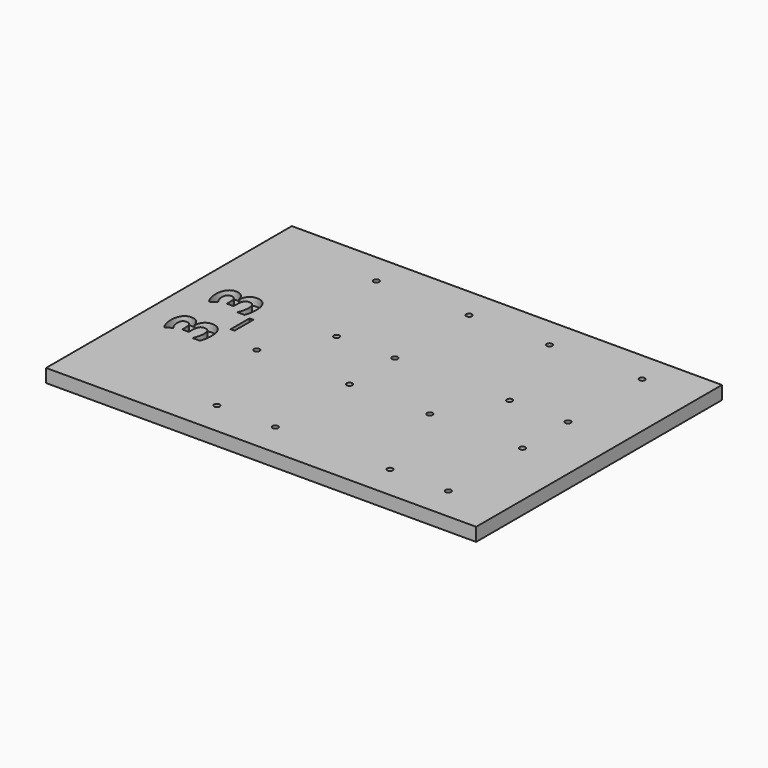
from build123d import *

# Parameters (mm, degrees)
F0_W         = 84
F0_H         = 60
F1_DEPTH     = 2.6
F2_TEXT_SIZE = 11.1111111111
F3_DEPTH     = 1.5
F4_R         = 0.55
F5_DEPTH     = 2.6


# Not quite as in the source:
# - Text() gives the source's letters only with a copy of the font that has no kerning and outlines rounded to 1/6400 em; it was checked with that copy


with BuildPart() as f1:
    # F0 (on Top) → F1 (new body)
    with BuildSketch(Plane.XY):
        with Locations((-1.1587231159, 8.3350909071)):
            Rectangle(F0_W, F0_H)
    extrude(amount=F1_DEPTH)

    # F2 (on face) → F3 (cut)
    with BuildSketch(Plane.XY.offset(2.6)):
        with Locations(Location((-30.1587231159, -0.4149090929), (0, 0, 90))):
            Text('3_3', F2_TEXT_SIZE, font='Open Sans', font_style=FontStyle.BOLD, text_align=(TextAlign.LEFT, TextAlign.BOTTOM))
    extrude(amount=-F3_DEPTH, mode=Mode.SUBTRACT)

    # F4 (on face) → F5 (cut, through all)
    with BuildSketch(Plane.XY.offset(2.6)):
        with Locations((-21.7587231159, 32.2350909071)):
            Circle(F4_R)
        with Locations((-3.6587231159, 32.2350909071)):
            Circle(F4_R)
        with Locations((-3.6587231159, 14.1350909071)):
            Circle(F4_R)
        with Locations((-15.0587231159, 14.1350909071)):
            Circle(F4_R)
        with Locations((18.7412768841, 14.1350909071)):
            Circle(F4_R)
        with Locations((12.0412768841, 32.2350909071)):
            Circle(F4_R)
        with Locations((30.1412768841, 32.2350909071)):
            Circle(F4_R)
        with Locations((30.1412768841, 14.1350909071)):
            Circle(F4_R)
        with Locations((30.1412768841, 3.0350909071)):
            Circle(F4_R)
        with Locations((12.0412768841, 3.0350909071)):
            Circle(F4_R)
        with Locations((-3.6587231159, 3.0350909071)):
            Circle(F4_R)
        with Locations((-21.7587231159, 3.0350909071)):
            Circle(F4_R)
        with Locations((-15.0587231159, -15.0649090929)):
            Circle(F4_R)
        with Locations((-3.6587231159, -15.0649090929)):
            Circle(F4_R)
        with Locations((30.1412768841, -15.0649090929)):
            Circle(F4_R)
        with Locations((18.7412768841, -15.0649090929)):
            Circle(F4_R)
    extrude(amount=-F5_DEPTH, mode=Mode.SUBTRACT)


solid = f1.part
